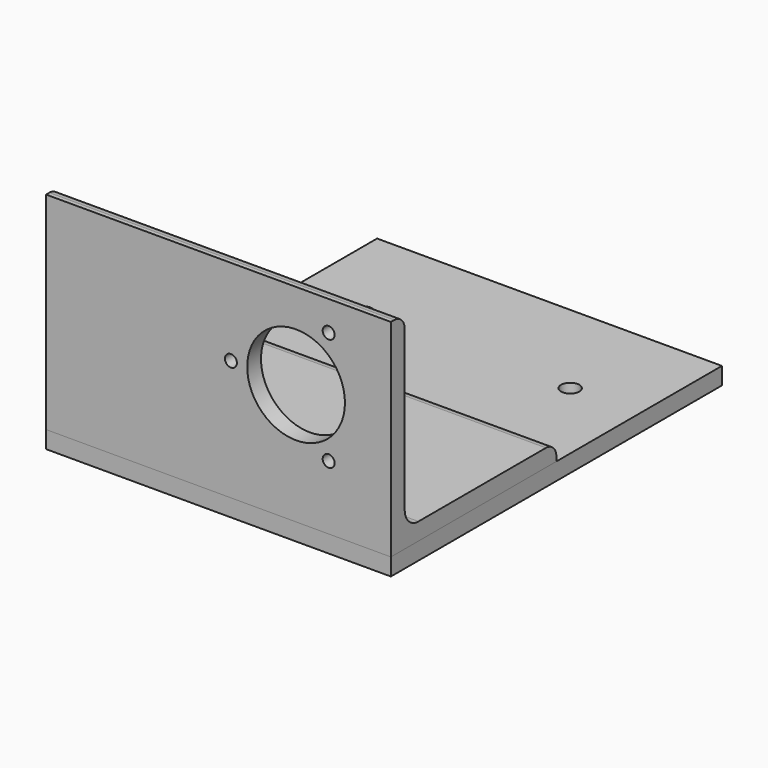
from build123d import *

# Parameters (mm, degrees)
F0_W      = 127
F0_H      = 152.4
F1_DEPTH  = 6.35
F3_D      = 6.746875
F3_DEPTH  = 10
F3_TIP    = 2.0269657445
F5_D      = 3.7973
F5_DEPTH  = 10
F5_TIP    = 1.1408240143
F7_DEPTH  = 63.5
F9_DEPTH  = 12.701
F10_R     = 18
F11_DEPTH = 25
F13_D     = 4.4


# Not quite as in the source:
# - a length typed as a fraction of an inch, garbled in the dataset ("3 / 203.2 mm" for 3/8 in), is restored


with BuildPart() as f1:
    # F0 (on Top) → F1 (new body)
    with BuildSketch(Plane.XY):
        Rectangle(F0_W, F0_H)
    extrude(amount=F1_DEPTH)

    # F3
    with Locations(Plane.XY.offset(6.35)):
        with Locations((-38.1, 38.1), (38.1, 38.1)):
            Hole(F3_D / 2, depth=F3_DEPTH)
            with Locations((0, 0, -(F3_DEPTH + F3_TIP / 2))):  # 118° drill point
                Cone(0, F3_D / 2, F3_TIP, mode=Mode.SUBTRACT)

    # F5
    with Locations(Plane.XY.offset(6.35)):
        with Locations((-47.625, -42.926), (-9.525, -42.926)):
            Hole(F5_D / 2, depth=F5_DEPTH)
            with Locations((0, 0, -(F5_DEPTH + F5_TIP / 2))):  # 118° drill point
                Cone(0, F5_D / 2, F5_TIP, mode=Mode.SUBTRACT)


with BuildPart() as f7:
    # F6 (on Right) → F7 (new body, symmetric)
    with BuildSketch(Plane.YZ):
        with BuildLine():
            Line((-76.2, 82.55), (-76.2, 6.35))
            Line((-76.2, 6.35), (0, 6.35))
            Line((0, 6.35), (0, 7.874))
            ThreePointArc((0, 7.874), (-1.413502674, 11.286497326), (-4.826, 12.7))
            Line((-4.826, 12.7), (-63.5, 12.7))
            ThreePointArc((-63.5, 12.7), (-67.9901280605, 14.5598719395), (-69.85, 19.05))
            Line((-69.85, 19.05), (-69.85, 77.724))
            ThreePointArc((-69.85, 77.724), (-71.263502674, 81.136497326), (-74.676, 82.55))
            Line((-74.676, 82.55), (-76.2, 82.55))
        make_face()
    extrude(amount=F7_DEPTH, both=True)

    # F8 (on face) → F9 (cut, through all)
    with BuildSketch(Plane.XY.offset(12.7)):
        with BuildLine():
            Line((-41.275, -39.624), (-53.975, -39.624))
            ThreePointArc((-53.975, -39.624), (-57.277, -42.926), (-53.975, -46.228))
            Line((-53.975, -46.228), (-41.275, -46.228))
            ThreePointArc((-41.275, -46.228), (-37.973, -42.926), (-41.275, -39.624))
        make_face()
        with BuildLine():
            Line((-3.175, -39.624), (-15.875, -39.624))
            ThreePointArc((-15.875, -39.624), (-19.177, -42.926), (-15.875, -46.228))
            Line((-15.875, -46.228), (-3.175, -46.228))
            ThreePointArc((-3.175, -46.228), (0.127, -42.926), (-3.175, -39.624))
        make_face()
    extrude(amount=-F9_DEPTH, mode=Mode.SUBTRACT)

    # F10 (on face) → F11 (cut)
    with BuildSketch(Plane.XZ.offset(76.2)):
        with Locations((28.575, 50.8)):
            Circle(F10_R)
    extrude(amount=-F11_DEPTH, mode=Mode.SUBTRACT)

    # F13 (through all)
    with Locations(Plane.XZ.offset(76.2)):
        with Locations((4.575, 50.8), (40.575, 71.5846096908), (40.575, 30.0153903092)):
            Hole(F13_D / 2)


solid = Compound([f1.part, f7.part])
